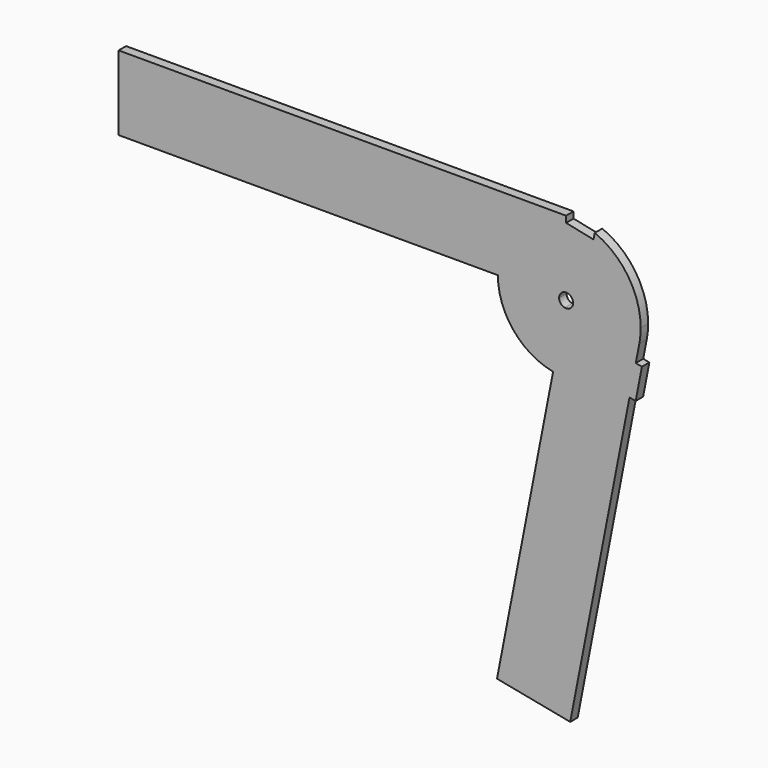
from build123d import *

# Parameters (mm, degrees)
F1_DEPTH = 6.35


with BuildPart() as f1:
    # F0 (on Front) → F1 (new body)
    with BuildSketch(Plane.XZ):
        with BuildLine():
            ThreePointArc((-50.8, 0), (-35.9210244843, 35.9210244843), (0, 50.8))
            Line((0, 50.8), (-304.8, 50.8))
            Line((-304.8, 50.8), (-304.8, 0))
            Line((-304.8, 0), (-50.8, 0))
        make_face()
        Polygon((51.6320080606, -22.9739477141), (46.3118022943, -27.9812591796), (43.1772616128, -44.1070730311), (47.3658829955, -44.9212585503), align=None)
        Polygon((51.6320080606, -22.9739477141), (47.4433866779, -22.1597621949), (46.3118022943, -27.9812591796), align=None)
        with BuildLine():
            Line((46.482, 0), (50.8, 0))
            ThreePointArc((50.8, 0), (42.2710462755, 28.1744325014), (19.5480847725, 46.8882968525))
            Line((19.5480847725, 46.8882968525), (18.6457425678, 42.5783114754))
            ThreePointArc((18.6457425678, 42.5783114754), (38.905447755, 25.4350635734), (46.482, 0))
        make_face()
        with BuildLine():
            Line((47.4433866779, -22.1597621949), (49.8666609191, -9.6930969651))
            ThreePointArc((49.8666609191, -9.6930969651), (28.4069994963, -42.1151086858), (-9.6930969651, -49.8666609191))
            Line((-9.6930969651, -49.8666609191), (-47.0680440019, -242.1440947937))
            Line((-47.0680440019, -242.1440947937), (2.7986169173, -251.8371917588))
            Line((2.7986169173, -251.8371917588), (43.1772616128, -44.1070730311))
            Line((43.1772616128, -44.1070730311), (46.3118022943, -27.9812591796))
            Line((46.3118022943, -27.9812591796), (47.4433866779, -22.1597621949))
        make_face()
        with BuildLine():
            ThreePointArc((49.8666609191, -9.6930969651), (50.5661268771, -4.868964228), (50.8, 0))
            Line((50.8, 0), (46.482, 0))
            ThreePointArc((46.482, 0), (46.2680060925, -4.4551022686), (45.627994741, -8.8691837231))
            Line((45.627994741, -8.8691837231), (49.8666609191, -9.6930969651))
        make_face()
        with BuildLine():
            Line((0, 46.482), (0, 50.8))
            ThreePointArc((0, 50.8), (-35.9210244843, 35.9210244843), (-50.8, 0))
            Line((-50.8, 0), (-46.482, 0))
            ThreePointArc((-46.482, 0), (-32.8677374031, 32.8677374031), (0, 46.482))
        make_face()
        with BuildLine():
            ThreePointArc((-9.6930969651, -49.8666609191), (28.4069994963, -42.1151086858), (49.8666609191, -9.6930969651))
            Line((49.8666609191, -9.6930969651), (45.627994741, -8.8691837231))
            ThreePointArc((45.627994741, -8.8691837231), (25.9924045391, -38.5353244475), (-8.8691837231, -45.627994741))
            Line((-8.8691837231, -45.627994741), (-9.6930969651, -49.8666609191))
        make_face()
        with BuildLine():
            Line((4.7625, 0), (46.482, 0))
            ThreePointArc((46.482, 0), (38.905447755, 25.4350635734), (18.6457425678, 42.5783114754))
            Line((18.6457425678, 42.5783114754), (0, 46.482))
            Line((0, 46.482), (0, 4.7625))
            ThreePointArc((0, 4.7625), (0.4564653964, 4.7405743947), (0.9087278405, 4.6749994612))
            ThreePointArc((0.9087278405, 4.6749994612), (3.6748620784, 3.0293225241), (4.7625, 0))
        make_face()
        with BuildLine():
            Line((0, 4.7625), (0, 46.482))
            ThreePointArc((0, 46.482), (-32.8677374031, 32.8677374031), (-46.482, 0))
            Line((-46.482, 0), (-4.7625, 0))
            ThreePointArc((-4.7625, 0), (-3.3675960454, 3.3675960454), (0, 4.7625))
        make_face()
        with BuildLine():
            ThreePointArc((-46.482, 0), (-35.866653885, -29.566187835), (-8.8691837231, -45.627994741))
            Line((-8.8691837231, -45.627994741), (-0.9087278405, -4.6749994612))
            ThreePointArc((-0.9087278405, -4.6749994612), (-3.6748620784, -3.0293225241), (-4.7625, 0))
            Line((-4.7625, 0), (-46.482, 0))
        make_face()
        with BuildLine():
            ThreePointArc((-8.8691837231, -45.627994741), (25.9924045391, -38.5353244475), (45.627994741, -8.8691837231))
            Line((45.627994741, -8.8691837231), (4.6749994612, -0.9087278405))
            ThreePointArc((4.6749994612, -0.9087278405), (2.6631562028, -3.9482914393), (-0.9087278405, -4.6749994612))
            Line((-0.9087278405, -4.6749994612), (-8.8691837231, -45.627994741))
        make_face()
        with BuildLine():
            ThreePointArc((45.627994741, -8.8691837231), (46.2680060925, -4.4551022686), (46.482, 0))
            Line((46.482, 0), (4.7625, 0))
            ThreePointArc((4.7625, 0), (4.7405743947, -0.4564653964), (4.6749994612, -0.9087278405))
            Line((4.6749994612, -0.9087278405), (45.627994741, -8.8691837231))
        make_face()
    extrude(amount=F1_DEPTH)


solid = f1.part
